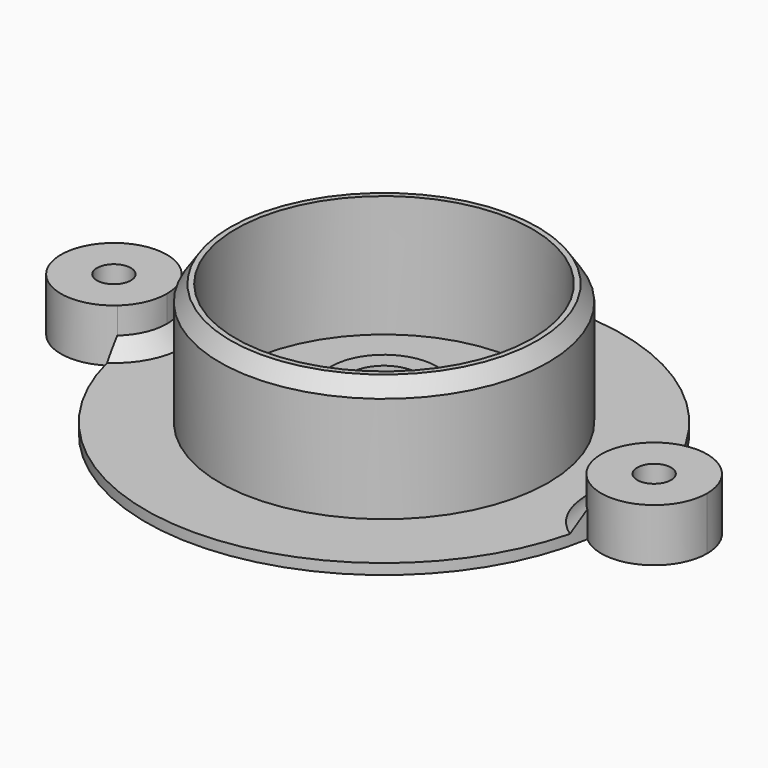
from build123d import *

# Parameters (mm, degrees)
F0_R         = 1.6
F1_DEPTH     = 5
F2_DEPTH     = 1
F3_R         = 15.5
F3_R_2       = 14
F4_DEPTH     = 11.5
F5_SIZE2     = 1.5
F5_SIZE      = 1
F8_T4_ANGLE  = 185.4300536725
F8_S5_R      = 22.5
F8_T6_DEPTH  = 9
F8_T10_ANGLE = 185.4300536725
F8_S11_R     = 22.5
F8_T12_DEPTH = 9
F9_R         = 5
F10_DEPTH    = 3
F11_R        = 3.25
F12_DEPTH    = 5


# Not quite as in the source:
# - a fillet or chamfer that OpenCascade refuses, or shapes differently, is made with other operations: its cross-section is extruded or revolved along the edge and cut away or added
# - a feature of the source that left no trace in its solid (it failed there, or was rolled back) is left out


with BuildPart() as f1:
    # F0 (on Top) → F1 (new body)
    with BuildSketch(Plane.XY):
        with BuildLine():
            ThreePointArc((-22.1862745098, -3.7442253372), (-22.5, 0), (-22.1862745098, 3.7442253372))
            ThreePointArc((-22.1862745098, 3.7442253372), (-30.5, 0), (-22.1862745098, -3.7442253372))
        make_face()
        with Locations((-25.5, 0)):
            Circle(F0_R, mode=Mode.SUBTRACT)
        with BuildLine():
            ThreePointArc((-20.5, 0), (-20.9410183456, 2.0532136456), (-22.1862745098, 3.7442253372))
            ThreePointArc((-22.1862745098, 3.7442253372), (-22.5, 0), (-22.1862745098, -3.7442253372))
            ThreePointArc((-22.1862745098, -3.7442253372), (-20.9410183456, -2.0532136456), (-20.5, 0))
        make_face()
    extrude(amount=F1_DEPTH)



with BuildPart() as f1b:
    # F0 (on Top) → F1, piece 2 (new body)
    with BuildSketch(Plane.XY):
        with BuildLine():
            ThreePointArc((22.1862745098, 3.7442253372), (22.4214314493, 1.8786728733), (22.5, 0))
            ThreePointArc((22.5, 0), (22.4214314493, -1.8786728733), (22.1862745098, -3.7442253372))
            ThreePointArc((22.1862745098, -3.7442253372), (27.5532136456, -4.5589816544), (30.5, 0))
            ThreePointArc((30.5, 0), (27.5532136456, 4.5589816544), (22.1862745098, 3.7442253372))
        make_face()
        with Locations((25.5, 0)):
            Circle(F0_R, mode=Mode.SUBTRACT)
        with BuildLine():
            ThreePointArc((22.1862745098, -3.7442253372), (22.4214314493, -1.8786728733), (22.5, 0))
            ThreePointArc((22.5, 0), (22.4214314493, 1.8786728733), (22.1862745098, 3.7442253372))
            ThreePointArc((22.1862745098, 3.7442253372), (20.5, 0), (22.1862745098, -3.7442253372))
        make_face()
    extrude(amount=F1_DEPTH)


with BuildPart() as f1_1:
    add(f1.part)

    add(f1b.part)  # F2 merges F1b
    # F0 (on Top) → F2 (join)
    with BuildSketch(Plane.XY):
        with BuildLine():
            ThreePointArc((22.1862745098, -3.7442253372), (20.5, 0), (22.1862745098, 3.7442253372))
            ThreePointArc((22.1862745098, 3.7442253372), (0, 22.5), (-22.1862745098, 3.7442253372))
            ThreePointArc((-22.1862745098, 3.7442253372), (-20.9410183456, 2.0532136456), (-20.5, 0))
            ThreePointArc((-20.5, 0), (-20.9410183456, -2.0532136456), (-22.1862745098, -3.7442253372))
            ThreePointArc((-22.1862745098, -3.7442253372), (0, -22.5), (22.1862745098, -3.7442253372))
        make_face()
    extrude(amount=F2_DEPTH)

    # F3 (on face) → F4 (join)
    with BuildSketch(Plane.XY.offset(1)):
        Circle(F3_R)
        Circle(F3_R_2, mode=Mode.SUBTRACT)
    extrude(amount=F4_DEPTH)

    # F5
    f5_edges = [f1_1.edges().sort_by_distance(p)[0] for p in [
        (-15.5, 0, 12.5),
    ]]
    f5_side = f1_1.faces().sort_by_distance((-15.061594, 0, 12.5))[0]
    chamfer(f5_edges, length=F5_SIZE, length2=F5_SIZE2, reference=f5_side)

    # F8: chamfer of 1.5 on 2 edges, made by hand


with BuildPart() as f8_tool2:
    # F8_s3 → F8_t4 (revolve)
    with BuildSketch(Plane(origin=(25.4427839223, 1.2065389767, 0), x_dir=(0, 0, 1), z_dir=(0.9988774861, 0.0473684257, 0))):
        Polygon((1, 7.7078948555), (2.5, 6.2078948555), (1, 6.2078948555), align=None)
    revolve(axis=Axis((25.5, 0, 1), (0, 0, -1)), revolution_arc=F8_T4_ANGLE)

    # F8_s5 → F8_t6 (intersect, symmetric)
    with BuildSketch(Plane.XY.offset(1.8)):
        Circle(F8_S5_R)
    extrude(amount=F8_T6_DEPTH, both=True, mode=Mode.INTERSECT)


with BuildPart() as f1_2:
    add(f1_1.part)

    # F8_t1: union F8_tool2
    add(f8_tool2.part)


with BuildPart() as f8_tool8:
    # F8_s9 → F8_t10 (revolve)
    with BuildSketch(Plane(origin=(-25.4427839223, 1.2065389767, 0), x_dir=(0, 0, 1), z_dir=(-0.9988774861, 0.0473684257, 0))):
        Polygon((1, -7.7078948555), (2.5, -6.2078948555), (1, -6.2078948555), align=None)
    revolve(axis=Axis((-25.5, 0, 1), (0, 0, 1)), revolution_arc=F8_T10_ANGLE)

    # F8_s11 → F8_t12 (intersect, symmetric)
    with BuildSketch(Plane.XY.offset(1.7)):
        Circle(F8_S11_R)
    extrude(amount=F8_T12_DEPTH, both=True, mode=Mode.INTERSECT)


with BuildPart() as f1_3:
    add(f1_2.part)

    # F8_t7: union F8_tool8
    add(f8_tool8.part)

    # F9 (on face) → F10 (join)
    with BuildSketch(Plane.XY.offset(1)):
        Circle(F9_R)
    extrude(amount=F10_DEPTH)

    # F11 (on face) → F12 (cut)
    with BuildSketch(Plane.XY.offset(4)):
        Circle(F11_R)
    extrude(amount=-F12_DEPTH, mode=Mode.SUBTRACT)


solid = f1_3.part
